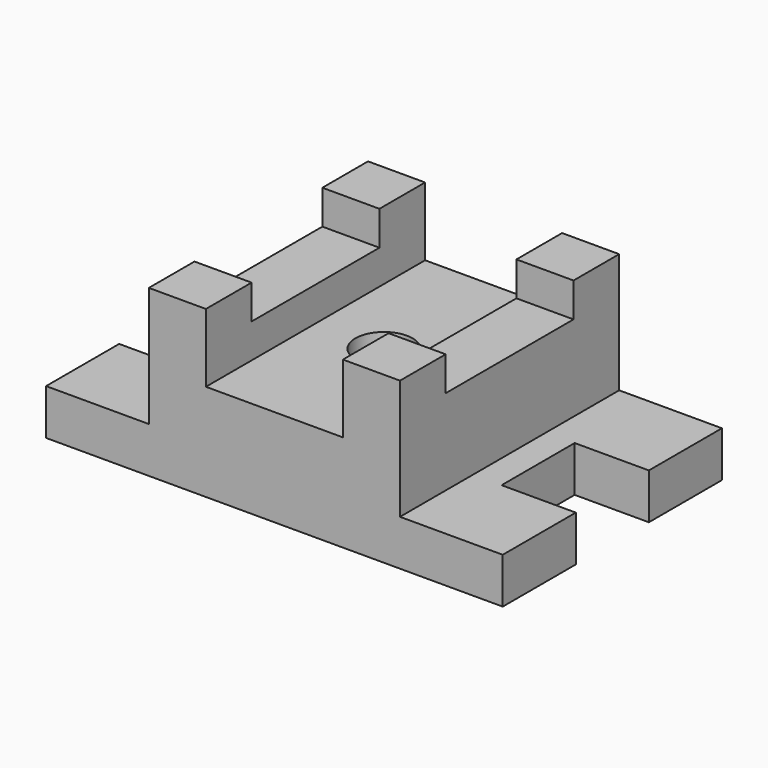
from build123d import *

# Parameters (mm, degrees)
F1_DEPTH = 25.4
F0_R     = 15.875
F2_DEPTH = 53.975
F0_W     = 31.75
F0_H     = 88.9
F3_DEPTH = 73.025
F0_H_2   = 31.75
F4_DEPTH = 92.075


# Not quite as in the source:
# - a feature names something its author has since deleted; it is built from what else it names


with BuildPart() as f1:
    # F0 (on Top) → F1 (new body)
    with BuildSketch(Plane.XY):
        Polygon((-75.5807677343, 77.5184368145), (-132.7307677343, 77.5184368145), (-132.7307677343, 26.7184368145), (-91.4557677343, 26.7184368145), (-91.4557677343, -24.0815631855), (-132.7307677343, -24.0815631855), (-132.7307677343, -74.8815631855), (-75.5807677344, -74.8815631855), (-75.5807677343, -43.1315631855), (-75.5807677343, 45.7684368145), align=None)
    extrude(amount=F1_DEPTH)



with BuildPart() as f1b:
    # F0 (on Top) → F1, piece 2 (new body)
    with BuildSketch(Plane.XY):
        Polygon((121.2692322657, 77.5184368145), (64.1192322657, 77.5184368145), (64.1192322657, 45.7684368145), (64.1192322657, -43.1315631855), (64.1192322657, -74.8815631855), (121.2692322657, -74.8815631855), (121.2692322657, -24.0815631855), (79.9942322657, -24.0815631855), (79.9942322657, 26.7184368145), (121.2692322657, 26.7184368145), align=None)
    extrude(amount=F1_DEPTH)


with BuildPart() as f2:
    # F0 (on Top) → F2 (new body)
    with BuildSketch(Plane.XY):
        Polygon((32.3692322657, 77.5184368145), (-43.8307677343, 77.5184368145), (-43.8307677343, 45.7684368145), (-43.8307677343, -43.1315631855), (-43.8307677343, -74.8815631855), (32.3692322657, -74.8815631855), (32.3692322657, -43.1315631855), (32.3692322657, 45.7684368145), align=None)
        with Locations((-5.7307677343, 1.3184368145)):
            Circle(F0_R, mode=Mode.SUBTRACT)
    extrude(amount=F2_DEPTH)


with BuildPart() as f1_1:
    add(f1.part)

    add(f1b.part)  # F3 merges F1b

    add(f2.part)  # F3 merges F2
    # F0 (on Top) → F3 (join)
    with BuildSketch(Plane.XY):
        with Locations((-59.7057677343, 1.3184368145)):
            Rectangle(F0_W, F0_H)
        with Locations((48.2442322657, 1.3184368145)):
            Rectangle(F0_W, F0_H)
    extrude(amount=F3_DEPTH)

    # F0 (on Top) → F4 (join)
    with BuildSketch(Plane.XY):
        with Locations((-59.7057677343, 61.6434368145)):
            Rectangle(F0_W, F0_H_2)
        with Locations((48.2442322657, 61.6434368145)):
            Rectangle(F0_W, F0_H_2)
        with Locations((-59.7057677343, -59.0065631855)):
            Rectangle(F0_W, F0_H_2)
        with Locations((48.2442322657, -59.0065631855)):
            Rectangle(F0_W, F0_H_2)
    extrude(amount=F4_DEPTH)


solid = f1_1.part
